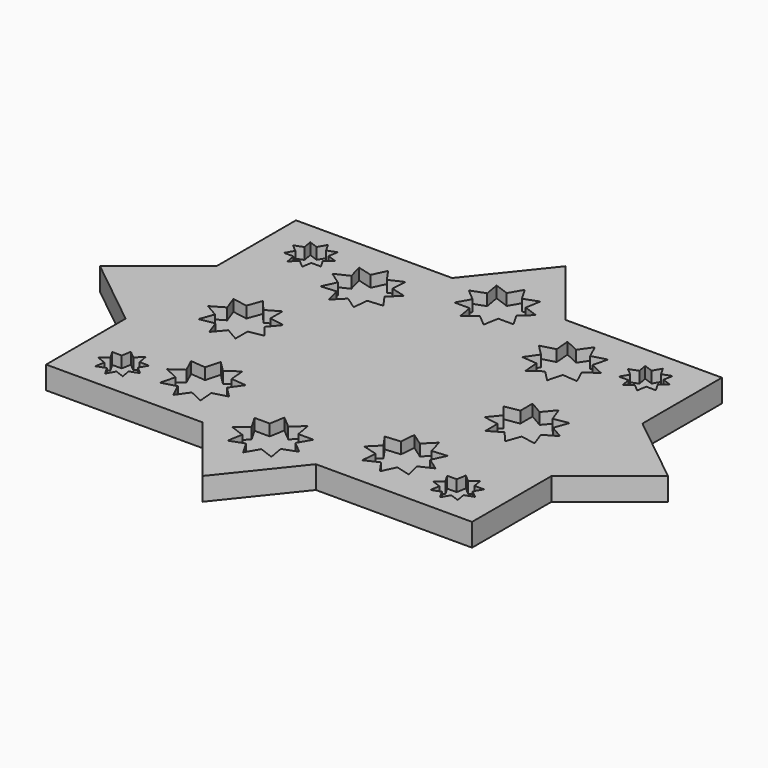
from build123d import *

# Parameters (mm, degrees)
F1_DEPTH          = 3
F3_DEPTH          = 25
F5_DEPTH          = 5
F8_DEPTH          = 4
F8_COPIES_COUNT   = 8
F10_DEPTH         = 4
F10_COPIES2_COUNT = 2


# Not quite as in the source:
# - a pattern or mirror of a feature is missing from the dataset's text; its kind, count and spacing are read off the source's solid


with BuildPart() as f1:
    # F0 (on Top) → F1 (new body)
    with BuildSketch(Plane.XY):
        Polygon((75, 20), (75, 55), (20, 55), (0, 80), (-20, 55), (-75, 55), (-75, 20), (-100, 0), (-75, -20), (-75, -55), (-20, -55), (0, -80), (20, -55), (75, -55), (75, -20), (100, 0), align=None)
    extrude(amount=F1_DEPTH)

    # F2 (on face) → F3 (cut)
    with BuildSketch(Plane.XY.offset(3)):
        Polygon((-57.3600895814, -2.6788535292), (-59.1925333174, -7.7134513162), (-53.916221868, -6.7830952491), (-52.083778132, -11.8176930361), (-48.6399104186, -7.7134513162), (-44, -10.3923048454), (-44, -5.0345977871), (-38.7236885506, -4.1042417199), (-42.167556264, 0), (-38.7236885506, 4.1042417199), (-44, 5.0345977871), (-44, 10.3923048454), (-48.6399104186, 7.7134513162), (-52.083778132, 11.8176930361), (-53.916221868, 6.7830952491), (-59.1925333174, 7.7134513162), (-57.3600895814, 2.6788535292), (-62, 0), align=None)
        Polygon((66.3602124411, -42.8563839129), (63.7950613662, -40.703966592), (65.4693448219, -37.8040225804), (62.1207779105, -37.8040225804), (61.5393053685, -34.5063279245), (58.9741542935, -36.6587452454), (56.4090032186, -34.5063279245), (55.8275306766, -37.8040225804), (52.4789637652, -37.8040225804), (54.1532472209, -40.703966592), (51.5880961459, -42.8563839129), (54.7347197629, -44.0016612479), (54.1532472209, -47.2993559038), (57.2998708378, -46.1540785688), (58.9741542935, -49.0540225804), (60.6484377493, -46.1540785688), (63.7950613662, -47.2993559038), (63.2135888242, -44.0016612479), align=None)
    extrude(amount=-F3_DEPTH, mode=Mode.SUBTRACT)

    # F4 (on face) → F5 (join)
    with BuildSketch(Plane(origin=(0, 0, 0), x_dir=(1, 0, 0), z_dir=(0, 0, -1))):
        Polygon((0, 80), (-20, 55), (-75, 55), (-75, 20), (-100, 0), (-75, -20), (-75, -55), (-20, -55), (0, -80), (20, -55), (75, -55), (75, -20), (100, 0), (75, 20), (75, 55), (20, 55), align=None)
    extrude(amount=F5_DEPTH)

    # F7 (on face) → F8 (cut)
    with BuildSketch(Plane.XY.offset(3)):
        Polygon((-44, -5.0345977871), (-38.7236885506, -4.1042417199), (-42.167556264, 0), (-38.7236885506, 4.1042417199), (-44, 5.0345977871), (-44, 10.3923048454), (-48.6399104186, 7.7134513162), (-52.083778132, 11.8176930361), (-53.916221868, 6.7830952491), (-59.1925333174, 7.7134513162), (-57.3600895814, 2.6788535292), (-62, 0), (-57.3600895814, -2.6788535292), (-59.1925333174, -7.7134513162), (-53.916221868, -6.7830952491), (-52.083778132, -11.8176930361), (-48.6399104186, -7.7134513162), (-44, -10.3923048454), align=None)
    f8 = extrude(amount=-F8_DEPTH, mode=Mode.SUBTRACT)

    # F8_copies: F8 ×8 about axis
    f8_copies_axis = Axis((0, 0, 0), (0, 0, 1))
    for i in range(1, F8_COPIES_COUNT):
        add(f8.rotate(f8_copies_axis, i * 360 / F8_COPIES_COUNT), mode=Mode.SUBTRACT)

    # F9 (on face) → F10 (cut)
    with BuildSketch(Plane.XY.offset(3)):
        Polygon((60.6484377493, -46.1540785688), (63.7950613662, -47.2993559038), (63.2135888242, -44.0016612479), (66.3602124411, -42.8563839129), (63.7950613662, -40.703966592), (65.4693448219, -37.8040225804), (62.1207779105, -37.8040225804), (61.5393053685, -34.5063279245), (58.9741542935, -36.6587452454), (56.4090032186, -34.5063279245), (55.8275306766, -37.8040225804), (52.4789637652, -37.8040225804), (54.1532472209, -40.703966592), (51.5880961459, -42.8563839129), (54.7347197629, -44.0016612479), (54.1532472209, -47.2993559038), (57.2998708378, -46.1540785688), (58.9741542935, -49.0540225804), align=None)
    f10 = extrude(amount=-F10_DEPTH, mode=Mode.SUBTRACT)

    # F10_copies: F10 across plane
    add(f10.mirror(Plane.ZX), mode=Mode.SUBTRACT)

    # F10_copies1: F10 across plane
    add(f10.mirror(Plane(origin=(0, 0, 0), x_dir=(0, 0, -1), z_dir=(-1, 0, 0))), mode=Mode.SUBTRACT)

    # F10_copies2: F10 ×2 about axis
    f10_copies2_axis = Axis((0, 0, 0), (0, 0, 1))
    for i in range(1, F10_COPIES2_COUNT):
        add(f10.rotate(f10_copies2_axis, i * 360 / F10_COPIES2_COUNT), mode=Mode.SUBTRACT)


solid = f1.part
